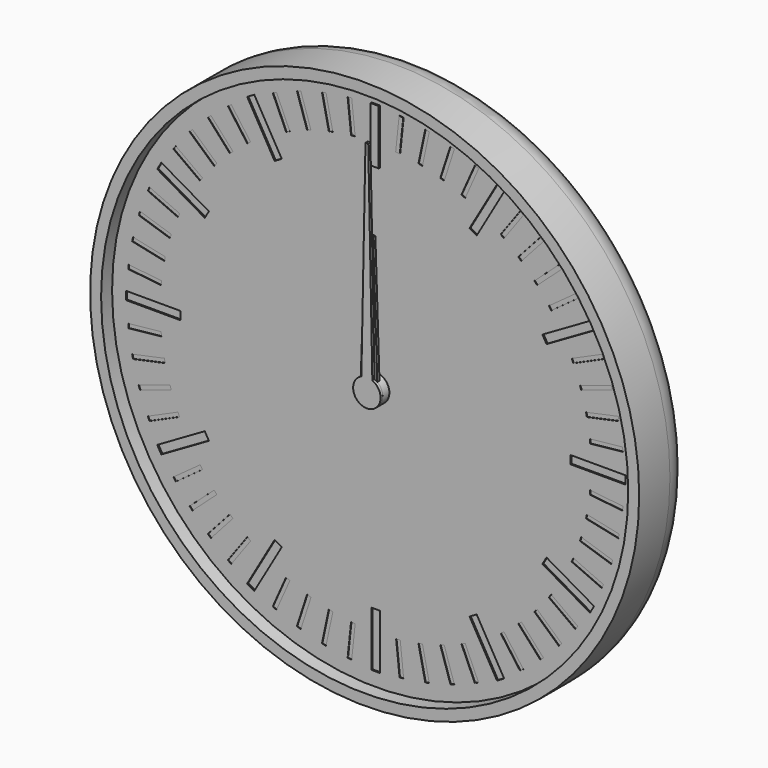
from build123d import *

# Parameters (mm, degrees)
F0_R      = 100
F1_DEPTH  = 24
F2_R      = 10
F3_T      = -4
F4_R      = 5
F4_R_2    = 3
F5_DEPTH  = 2
F6_DEPTH  = 19
F7_DEPTH  = 8
F9_DEPTH  = 4
F11_DEPTH = 4
F12_R     = 5
F12_R_2   = 3
F13_DEPTH = 2
F14_R     = 3
F15_DEPTH = 4
F17_DEPTH = 4
F18_R     = 3
F19_DEPTH = 2
F20_R     = 98
F20_R_2   = 5
F21_DEPTH = 1
F23_R     = 5
F23_R_2   = 3
F24_DEPTH = 2
F25_W     = 3
F25_H     = 20
F25_W_2   = 20
F25_H_2   = 3
F26_DEPTH = 0.5
F27_W     = 1.5
F27_H     = 12
F27_W_2   = 12
F27_H_2   = 1.5
F28_DEPTH = 0.2
F29_DEPTH = 1
F30_DEPTH = 0.4
F31_R     = 5
F31_R_2   = 3
F32_DEPTH = 5
F33_R     = 3
F34_DEPTH = 1
F36_DEPTH = 1


with BuildPart() as f1:
    # F0 (on Front) → F1 (new body)
    with BuildSketch(Plane.XZ):
        Circle(F0_R)
    extrude(amount=F1_DEPTH)

    # F2
    f2_edges = [f1.edges().sort_by_distance(p)[0] for p in [
        (-100, 0, 0),
    ]]
    fillet(f2_edges, radius=F2_R)

    # F3
    f3_openings = [f1.faces().sort_by_distance(p)[0] for p in [
        (0, -24, 0),
    ]]
    offset(amount=F3_T, openings=f3_openings)

    # F4 (on face) → F5 (join)
    with BuildSketch(Plane.XZ.offset(4)):
        Circle(F4_R)
        Circle(F4_R_2, mode=Mode.SUBTRACT)
        with Locations((40, 0)):
            Circle(F4_R)
        with Locations((40, 0)):
            Circle(F4_R_2, mode=Mode.SUBTRACT)
    extrude(amount=F5_DEPTH)


with BuildPart() as f6:
    # F6 (new): a face of the model
    f6_faces = [f1.part.faces().sort_by_distance(p)[0] for p in [
        (0, -4, 0),
    ]]
    extrude(f6_faces, amount=F6_DEPTH)

    # F8 (on face) → F9 (join)
    with BuildSketch(Plane.XZ.offset(6)):
        with BuildLine():
            ThreePointArc((9.2729637667, -1.3794085621), (9.3494561423, -0.6915886375), (9.375, 0))
            ThreePointArc((9.375, 0), (9.3494561423, 0.6915886375), (9.2729637667, 1.3794085621))
            ThreePointArc((9.2729637667, 1.3794085621), (8.9161548403, 2.8970343223), (8.3127812852, 4.3345463782))
            ThreePointArc((8.3127812852, 4.3345463782), (7.5845343223, 5.5104867402), (6.6911892658, 6.566476316))
            ThreePointArc((6.6911892658, 6.566476316), (5.5104867402, 7.5845343223), (4.1773988938, 8.3928519278))
            ThreePointArc((4.1773988938, 8.3928519278), (2.8970343223, 8.9161548403), (1.5536078905, 9.2453733036))
            ThreePointArc((1.5536078905, 9.2453733036), (0, 9.375), (-1.5536078905, 9.2453733036))
            ThreePointArc((-1.5536078905, 9.2453733036), (-2.8970343223, 8.9161548403), (-4.1773988938, 8.3928519278))
            ThreePointArc((-4.1773988938, 8.3928519278), (-5.5104867402, 7.5845343223), (-6.6911892658, 6.566476316))
            ThreePointArc((-6.6911892658, 6.566476316), (-7.5845343223, 5.5104867402), (-8.3127812852, 4.3345463782))
            ThreePointArc((-8.3127812852, 4.3345463782), (-8.9161548403, 2.8970343223), (-9.2729637667, 1.3794085621))
            ThreePointArc((-9.2729637667, 1.3794085621), (-9.375, 0), (-9.2729637667, -1.3794085621))
            ThreePointArc((-9.2729637667, -1.3794085621), (-8.9161548403, -2.8970343223), (-8.3127812852, -4.3345463782))
            ThreePointArc((-8.3127812852, -4.3345463782), (-7.5845343223, -5.5104867402), (-6.6911892658, -6.566476316))
            ThreePointArc((-6.6911892658, -6.566476316), (-5.5104867402, -7.5845343223), (-4.1773988938, -8.3928519278))
            ThreePointArc((-4.1773988938, -8.3928519278), (-2.8970343223, -8.9161548403), (-1.5536078905, -9.2453733036))
            ThreePointArc((-1.5536078905, -9.2453733036), (0, -9.375), (1.5536078905, -9.2453733036))
            ThreePointArc((1.5536078905, -9.2453733036), (2.8970343223, -8.9161548403), (4.1773988938, -8.3928519278))
            ThreePointArc((4.1773988938, -8.3928519278), (5.5104867402, -7.5845343223), (6.6911892658, -6.566476316))
            ThreePointArc((6.6911892658, -6.566476316), (7.5845343223, -5.5104867402), (8.3127812852, -4.3345463782))
            ThreePointArc((8.3127812852, -4.3345463782), (8.9161548403, -2.8970343223), (9.2729637667, -1.3794085621))
        make_face()
        with BuildLine():
            ThreePointArc((8.3127812852, 4.3345463782), (8.9161548403, 2.8970343223), (9.2729637667, 1.3794085621))
            Line((9.2729637667, 1.3794085621), (11.1823199426, 2.3946312492))
            Line((11.1823199426, 2.3946312492), (10.8182678729, 3.515068311))
            Line((10.8182678729, 3.515068311), (10.4542158031, 4.6355053728))
            Line((10.4542158031, 4.6355053728), (8.3127812852, 4.3345463782))
        make_face()
        with BuildLine():
            Line((11.1823199426, -2.3946312492), (9.2729637667, -1.3794085621))
            ThreePointArc((9.2729637667, -1.3794085621), (8.9161548403, -2.8970343223), (8.3127812852, -4.3345463782))
            Line((8.3127812852, -4.3345463782), (10.4542158031, -4.6355053728))
            Line((10.4542158031, -4.6355053728), (10.8182678729, -3.515068311))
            Line((10.8182678729, -3.515068311), (11.1823199426, -2.3946312492))
        make_face()
        with BuildLine():
            ThreePointArc((4.1773988938, 8.3928519278), (5.5104867402, 7.5845343223), (6.6911892658, 6.566476316))
            Line((6.6911892658, 6.566476316), (7.6391579371, 8.5101001246))
            Line((7.6391579371, 8.5101001246), (6.6860572448, 9.202568311))
            Line((6.6860572448, 9.202568311), (5.7329565525, 9.8950364974))
            Line((5.7329565525, 9.8950364974), (4.1773988938, 8.3928519278))
        make_face()
        with BuildLine():
            Line((7.6391579371, -8.5101001246), (6.6911892658, -6.566476316))
            ThreePointArc((6.6911892658, -6.566476316), (5.5104867402, -7.5845343223), (4.1773988938, -8.3928519278))
            Line((4.1773988938, -8.3928519278), (5.7329565525, -9.8950364974))
            Line((5.7329565525, -9.8950364974), (6.6860572448, -9.202568311))
            Line((6.6860572448, -9.202568311), (7.6391579371, -8.5101001246))
        make_face()
        with BuildLine():
            ThreePointArc((-1.5536078905, 9.2453733036), (0, 9.375), (1.5536078905, 9.2453733036))
            Line((1.5536078905, 9.2453733036), (1.1780972451, 11.375))
            Line((1.1780972451, 11.375), (0, 11.375))
            Line((0, 11.375), (-1.1780972451, 11.375))
            Line((-1.1780972451, 11.375), (-1.5536078905, 9.2453733036))
        make_face()
        with BuildLine():
            Line((1.1780972451, -11.375), (1.5536078905, -9.2453733036))
            ThreePointArc((1.5536078905, -9.2453733036), (0, -9.375), (-1.5536078905, -9.2453733036))
            Line((-1.5536078905, -9.2453733036), (-1.1780972451, -11.375))
            Line((-1.1780972451, -11.375), (0, -11.375))
            Line((0, -11.375), (1.1780972451, -11.375))
        make_face()
        with BuildLine():
            ThreePointArc((-6.6911892658, 6.566476316), (-5.5104867402, 7.5845343223), (-4.1773988938, 8.3928519278))
            Line((-4.1773988938, 8.3928519278), (-5.7329565525, 9.8950364974))
            Line((-5.7329565525, 9.8950364974), (-6.6860572448, 9.202568311))
            Line((-6.6860572448, 9.202568311), (-7.6391579371, 8.5101001246))
            Line((-7.6391579371, 8.5101001246), (-6.6911892658, 6.566476316))
        make_face()
        with BuildLine():
            Line((-5.7329565525, -9.8950364974), (-4.1773988938, -8.3928519278))
            ThreePointArc((-4.1773988938, -8.3928519278), (-5.5104867402, -7.5845343223), (-6.6911892658, -6.566476316))
            Line((-6.6911892658, -6.566476316), (-7.6391579371, -8.5101001246))
            Line((-7.6391579371, -8.5101001246), (-6.6860572448, -9.202568311))
            Line((-6.6860572448, -9.202568311), (-5.7329565525, -9.8950364974))
        make_face()
        with BuildLine():
            ThreePointArc((-9.2729637667, 1.3794085621), (-8.9161548403, 2.8970343223), (-8.3127812852, 4.3345463782))
            Line((-8.3127812852, 4.3345463782), (-10.4542158031, 4.6355053728))
            Line((-10.4542158031, 4.6355053728), (-10.8182678729, 3.515068311))
            Line((-10.8182678729, 3.515068311), (-11.1823199426, 2.3946312492))
            Line((-11.1823199426, 2.3946312492), (-9.2729637667, 1.3794085621))
        make_face()
        with BuildLine():
            Line((-10.4542158031, -4.6355053728), (-8.3127812852, -4.3345463782))
            ThreePointArc((-8.3127812852, -4.3345463782), (-8.9161548403, -2.8970343223), (-9.2729637667, -1.3794085621))
            Line((-9.2729637667, -1.3794085621), (-11.1823199426, -2.3946312492))
            Line((-11.1823199426, -2.3946312492), (-10.8182678729, -3.515068311))
            Line((-10.8182678729, -3.515068311), (-10.4542158031, -4.6355053728))
        make_face()
    extrude(amount=F9_DEPTH)

    # F35 (on face) → F36 (join)
    with BuildSketch(Plane.XZ.offset(23)):
        with BuildLine():
            ThreePointArc((-2, 4.582575695), (-2.7386127875, -4.1833001327), (5, 0))
            ThreePointArc((5, 0), (4.1833001327, 2.7386127875), (2, 4.582575695))
            ThreePointArc((2, 4.582575695), (0, 5), (-2, 4.582575695))
        make_face()
        with BuildLine():
            ThreePointArc((-2, 4.582575695), (0, 5), (2, 4.582575695))
            Line((2, 4.582575695), (0.5, 80))
            Line((0.5, 80), (0, 80))
            Line((0, 80), (-0.5, 80))
            Line((-0.5, 80), (-2, 4.582575695))
        make_face()
    extrude(amount=-F36_DEPTH)


with BuildPart() as f7:
    # F7 (new): a face of the model
    f7_faces = [f1.part.faces().sort_by_distance(p)[0] for p in [
        (40, -4, 0),
    ]]
    extrude(f7_faces, amount=F7_DEPTH)

    # F10 (on face) → F11 (join)
    with BuildSketch(Plane.XZ.offset(6)):
        with BuildLine():
            ThreePointArc((68.0829066802, -1.5381733945), (68.1144747006, -0.7693746225), (68.125, 0))
            ThreePointArc((68.125, 0), (68.1144747006, 0.7693746225), (68.0829066802, 1.5381733945))
            ThreePointArc((68.0829066802, 1.5381733945), (67.9709283072, 2.9398630294), (67.7890320221, 4.3342039956))
            ThreePointArc((67.7890320221, 4.3342039956), (67.5104012706, 5.8475163042), (67.1494235596, 7.3433252263))
            ThreePointArc((67.1494235596, 7.3433252263), (66.7484645208, 8.6911029668), (66.280643318, 10.0171558733))
            ThreePointArc((66.280643318, 10.0171558733), (65.6934659962, 11.4394680865), (65.0293803521, 12.8275385085))
            ThreePointArc((65.0293803521, 12.8275385085), (64.3569644814, 14.0625), (63.6236643925, 15.2623099717))
            ThreePointArc((63.6236643925, 15.2623099717), (62.7536029668, 16.5314602207), (61.815433119, 17.7511268046))
            ThreePointArc((61.815433119, 17.7511268046), (60.9009482166, 18.8192983038), (59.934217974, 19.8404278876))
            ThreePointArc((59.934217974, 19.8404278876), (58.8192983038, 20.9009482166), (57.6480467764, 21.8989056799))
            ThreePointArc((57.6480467764, 21.8989056799), (56.5314602207, 22.7536029668), (55.3735505752, 23.5514238999))
            ThreePointArc((55.3735505752, 23.5514238999), (54.0625, 24.3569644814), (52.709356105, 25.0895972944))
            ThreePointArc((52.709356105, 25.0895972944), (51.4394680865, 25.6934659962), (50.1409852457, 26.2331096755))
            ThreePointArc((50.1409852457, 26.2331096755), (48.6911029668, 26.7484645208), (47.2152055856, 27.1837531139))
            ThreePointArc((47.2152055856, 27.1837531139), (45.8475163042, 27.5104012706), (44.4652101991, 27.7682826779))
            ThreePointArc((44.4652101991, 27.7682826779), (42.9398630294, 27.9709283072), (41.4057159597, 28.0898484802))
            ThreePointArc((41.4057159597, 28.0898484802), (40, 28.125), (38.5942840403, 28.0898484802))
            ThreePointArc((38.5942840403, 28.0898484802), (37.0601369706, 27.9709283072), (35.5347898009, 27.7682826779))
            ThreePointArc((35.5347898009, 27.7682826779), (34.1524836958, 27.5104012706), (32.7847944144, 27.1837531139))
            ThreePointArc((32.7847944144, 27.1837531139), (31.3088970332, 26.7484645208), (29.8590147543, 26.2331096755))
            ThreePointArc((29.8590147543, 26.2331096755), (28.5605319135, 25.6934659962), (27.290643895, 25.0895972944))
            ThreePointArc((27.290643895, 25.0895972944), (25.9375, 24.3569644814), (24.6264494248, 23.5514238999))
            ThreePointArc((24.6264494248, 23.5514238999), (23.4685397793, 22.7536029668), (22.3519532236, 21.8989056799))
            ThreePointArc((22.3519532236, 21.8989056799), (21.1807016962, 20.9009482166), (20.065782026, 19.8404278876))
            ThreePointArc((20.065782026, 19.8404278876), (19.0990517834, 18.8192983038), (18.184566881, 17.7511268046))
            ThreePointArc((18.184566881, 17.7511268046), (17.2463970332, 16.5314602207), (16.3763356075, 15.2623099717))
            ThreePointArc((16.3763356075, 15.2623099717), (15.6430355186, 14.0625), (14.9706196479, 12.8275385085))
            ThreePointArc((14.9706196479, 12.8275385085), (14.3065340038, 11.4394680865), (13.719356682, 10.0171558733))
            ThreePointArc((13.719356682, 10.0171558733), (13.2515354792, 8.6911029668), (12.8505764404, 7.3433252263))
            ThreePointArc((12.8505764404, 7.3433252263), (12.4895987294, 5.8475163042), (12.2109679779, 4.3342039956))
            ThreePointArc((12.2109679779, 4.3342039956), (12.0290716928, 2.9398630294), (11.9170933198, 1.5381733945))
            ThreePointArc((11.9170933198, 1.5381733945), (11.875, 0), (11.9170933198, -1.5381733945))
            ThreePointArc((11.9170933198, -1.5381733945), (12.0290716928, -2.9398630294), (12.2109679779, -4.3342039956))
            ThreePointArc((12.2109679779, -4.3342039956), (12.4895987294, -5.8475163042), (12.8505764404, -7.3433252263))
            ThreePointArc((12.8505764404, -7.3433252263), (13.2515354792, -8.6911029668), (13.719356682, -10.0171558733))
            ThreePointArc((13.719356682, -10.0171558733), (14.3065340038, -11.4394680865), (14.9706196479, -12.8275385085))
            ThreePointArc((14.9706196479, -12.8275385085), (15.6430355186, -14.0625), (16.3763356075, -15.2623099717))
            ThreePointArc((16.3763356075, -15.2623099717), (17.2463970332, -16.5314602207), (18.184566881, -17.7511268046))
            ThreePointArc((18.184566881, -17.7511268046), (19.0990517834, -18.8192983038), (20.065782026, -19.8404278876))
            ThreePointArc((20.065782026, -19.8404278876), (21.1807016962, -20.9009482166), (22.3519532236, -21.8989056799))
            ThreePointArc((22.3519532236, -21.8989056799), (23.4685397793, -22.7536029668), (24.6264494248, -23.5514238999))
            ThreePointArc((24.6264494248, -23.5514238999), (25.9375, -24.3569644814), (27.290643895, -25.0895972944))
            ThreePointArc((27.290643895, -25.0895972944), (28.5605319135, -25.6934659962), (29.8590147543, -26.2331096755))
            ThreePointArc((29.8590147543, -26.2331096755), (31.3088970332, -26.7484645208), (32.7847944144, -27.1837531139))
            ThreePointArc((32.7847944144, -27.1837531139), (34.1524836958, -27.5104012706), (35.5347898009, -27.7682826779))
            ThreePointArc((35.5347898009, -27.7682826779), (37.0601369706, -27.9709283072), (38.5942840403, -28.0898484802))
            ThreePointArc((38.5942840403, -28.0898484802), (40, -28.125), (41.4057159597, -28.0898484802))
            ThreePointArc((41.4057159597, -28.0898484802), (42.9398630294, -27.9709283072), (44.4652101991, -27.7682826779))
            ThreePointArc((44.4652101991, -27.7682826779), (45.8475163042, -27.5104012706), (47.2152055856, -27.1837531139))
            ThreePointArc((47.2152055856, -27.1837531139), (48.6911029668, -26.7484645208), (50.1409852457, -26.2331096755))
            ThreePointArc((50.1409852457, -26.2331096755), (51.4394680865, -25.6934659962), (52.709356105, -25.0895972944))
            ThreePointArc((52.709356105, -25.0895972944), (54.0625, -24.3569644814), (55.3735505752, -23.5514238999))
            ThreePointArc((55.3735505752, -23.5514238999), (56.5314602207, -22.7536029668), (57.6480467764, -21.8989056799))
            ThreePointArc((57.6480467764, -21.8989056799), (58.8192983038, -20.9009482166), (59.934217974, -19.8404278876))
            ThreePointArc((59.934217974, -19.8404278876), (60.9009482166, -18.8192983038), (61.815433119, -17.7511268046))
            ThreePointArc((61.815433119, -17.7511268046), (62.7536029668, -16.5314602207), (63.6236643925, -15.2623099717))
            ThreePointArc((63.6236643925, -15.2623099717), (64.3569644814, -14.0625), (65.0293803521, -12.8275385085))
            ThreePointArc((65.0293803521, -12.8275385085), (65.6934659962, -11.4394680865), (66.280643318, -10.0171558733))
            ThreePointArc((66.280643318, -10.0171558733), (66.7484645208, -8.6911029668), (67.1494235596, -7.3433252263))
            ThreePointArc((67.1494235596, -7.3433252263), (67.5104012706, -5.8475163042), (67.7890320221, -4.3342039956))
            ThreePointArc((67.7890320221, -4.3342039956), (67.9709283072, -2.9398630294), (68.0829066802, -1.5381733945))
        make_face()
        with BuildLine():
            ThreePointArc((68.0829066802, 1.5381733945), (68.1144747006, 0.7693746225), (68.125, 0))
            ThreePointArc((68.125, 0), (68.1144747006, -0.7693746225), (68.0829066802, -1.5381733945))
            Line((68.0829066802, -1.5381733945), (70.125, -1.1780972451))
            Line((70.125, -1.1780972451), (70.125, 0))
            Line((70.125, 0), (70.125, 1.1780972451))
            Line((70.125, 1.1780972451), (68.0829066802, 1.5381733945))
        make_face()
        with BuildLine():
            ThreePointArc((67.1494235596, 7.3433252263), (67.5104012706, 5.8475163042), (67.7890320221, 4.3342039956))
            Line((67.7890320221, 4.3342039956), (69.7116366623, 5.1109866922))
            Line((69.7116366623, 5.1109866922), (69.4666964721, 6.2633396859))
            Line((69.4666964721, 6.2633396859), (69.2217562819, 7.4156926796))
            Line((69.2217562819, 7.4156926796), (67.1494235596, 7.3433252263))
        make_face()
        with BuildLine():
            Line((69.7116366623, -5.1109866922), (67.7890320221, -4.3342039956))
            ThreePointArc((67.7890320221, -4.3342039956), (67.5104012706, -5.8475163042), (67.1494235596, -7.3433252263))
            Line((67.1494235596, -7.3433252263), (69.2217562819, -7.4156926796))
            Line((69.2217562819, -7.4156926796), (69.4666964721, -6.2633396859))
            Line((69.4666964721, -6.2633396859), (69.7116366623, -5.1109866922))
        make_face()
        with BuildLine():
            ThreePointArc((65.0293803521, 12.8275385085), (65.6934659962, 11.4394680865), (66.280643318, 10.0171558733))
            Line((66.280643318, 10.0171558733), (67.9997322302, 11.1766959857))
            Line((67.9997322302, 11.1766959857), (67.5205569115, 12.2529413727))
            Line((67.5205569115, 12.2529413727), (67.0413815928, 13.3291867596))
            Line((67.0413815928, 13.3291867596), (65.0293803521, 12.8275385085))
        make_face()
        with BuildLine():
            Line((67.9997322302, -11.1766959857), (66.280643318, -10.0171558733))
            ThreePointArc((66.280643318, -10.0171558733), (65.6934659962, -11.4394680865), (65.0293803521, -12.8275385085))
            Line((65.0293803521, -12.8275385085), (67.0413815928, -13.3291867596))
            Line((67.0413815928, -13.3291867596), (67.5205569115, -12.2529413727))
            Line((67.5205569115, -12.2529413727), (67.9997322302, -11.1766959857))
        make_face()
        with BuildLine():
            ThreePointArc((61.815433119, 17.7511268046), (62.7536029668, 16.5314602207), (63.6236643925, 15.2623099717))
            Line((63.6236643925, 15.2623099717), (65.064105142, 16.753930033))
            Line((65.064105142, 16.753930033), (64.3716369555, 17.7070307253))
            Line((64.3716369555, 17.7070307253), (63.6791687691, 18.6601314176))
            Line((63.6791687691, 18.6601314176), (61.815433119, 17.7511268046))
        make_face()
        with BuildLine():
            Line((65.064105142, -16.753930033), (63.6236643925, -15.2623099717))
            ThreePointArc((63.6236643925, -15.2623099717), (62.7536029668, -16.5314602207), (61.815433119, -17.7511268046))
            Line((61.815433119, -17.7511268046), (63.6791687691, -18.6601314176))
            Line((63.6791687691, -18.6601314176), (64.3716369555, -17.7070307253))
            Line((64.3716369555, -17.7070307253), (65.064105142, -16.753930033))
        make_face()
        with BuildLine():
            ThreePointArc((57.6480467764, 21.8989056799), (58.8192983038, 20.9009482166), (59.934217974, 19.8404278876))
            Line((59.934217974, 19.8404278876), (61.0330563882, 21.5989369435))
            Line((61.0330563882, 21.5989369435), (60.1575595166, 22.3872378675))
            Line((60.1575595166, 22.3872378675), (59.282062645, 23.1755387915))
            Line((59.282062645, 23.1755387915), (57.6480467764, 21.8989056799))
        make_face()
        with BuildLine():
            Line((61.0330563882, -21.5989369435), (59.934217974, -19.8404278876))
            ThreePointArc((59.934217974, -19.8404278876), (58.8192983038, -20.9009482166), (57.6480467764, -21.8989056799))
            Line((57.6480467764, -21.8989056799), (59.282062645, -23.1755387915))
            Line((59.282062645, -23.1755387915), (60.1575595166, -22.3872378675))
            Line((60.1575595166, -22.3872378675), (61.0330563882, -21.5989369435))
        make_face()
        with BuildLine():
            ThreePointArc((52.709356105, 25.0895972944), (54.0625, 24.3569644814), (55.3735505752, 23.5514238999))
            Line((55.3735505752, 23.5514238999), (56.0827621424, 25.4999666665))
            Line((56.0827621424, 25.4999666665), (55.0625, 26.089015289))
            Line((55.0625, 26.089015289), (54.0422378576, 26.6780639116))
            Line((54.0422378576, 26.6780639116), (52.709356105, 25.0895972944))
        make_face()
        with BuildLine():
            Line((56.0827621424, -25.4999666665), (55.3735505752, -23.5514238999))
            ThreePointArc((55.3735505752, -23.5514238999), (54.0625, -24.3569644814), (52.709356105, -25.0895972944))
            Line((52.709356105, -25.0895972944), (54.0422378576, -26.6780639116))
            Line((54.0422378576, -26.6780639116), (55.0625, -26.089015289))
            Line((55.0625, -26.089015289), (56.0827621424, -25.4999666665))
        make_face()
        with BuildLine():
            ThreePointArc((47.2152055856, 27.1837531139), (48.6911029668, 26.7484645208), (50.1409852457, 26.2331096755))
            Line((50.1409852457, 26.2331096755), (50.4295740173, 28.2865254836))
            Line((50.4295740173, 28.2865254836), (49.3091369555, 28.6505775534))
            Line((49.3091369555, 28.6505775534), (48.1886998938, 29.0146296232))
            Line((48.1886998938, 29.0146296232), (47.2152055856, 27.1837531139))
        make_face()
        with BuildLine():
            Line((50.4295740173, -28.2865254836), (50.1409852457, -26.2331096755))
            ThreePointArc((50.1409852457, -26.2331096755), (48.6911029668, -26.7484645208), (47.2152055856, -27.1837531139))
            Line((47.2152055856, -27.1837531139), (48.1886998938, -29.0146296232))
            Line((48.1886998938, -29.0146296232), (49.3091369555, -28.6505775534))
            Line((49.3091369555, -28.6505775534), (50.4295740173, -28.2865254836))
        make_face()
        with BuildLine():
            ThreePointArc((41.4057159597, 28.0898484802), (42.9398630294, 27.9709283072), (44.4652101991, 27.7682826779))
            Line((44.4652101991, 27.7682826779), (44.3205634611, 29.8368274034))
            Line((44.3205634611, 29.8368274034), (43.1489199559, 29.959972098))
            Line((43.1489199559, 29.959972098), (41.9772764508, 30.0831167926))
            Line((41.9772764508, 30.0831167926), (41.4057159597, 28.0898484802))
        make_face()
        with BuildLine():
            Line((44.3205634611, -29.8368274034), (44.4652101991, -27.7682826779))
            ThreePointArc((44.4652101991, -27.7682826779), (42.9398630294, -27.9709283072), (41.4057159597, -28.0898484802))
            Line((41.4057159597, -28.0898484802), (41.9772764508, -30.0831167926))
            Line((41.9772764508, -30.0831167926), (43.1489199559, -29.959972098))
            Line((43.1489199559, -29.959972098), (44.3205634611, -29.8368274034))
        make_face()
        with BuildLine():
            ThreePointArc((35.5347898009, 27.7682826779), (37.0601369706, 27.9709283072), (38.5942840403, 28.0898484802))
            Line((38.5942840403, 28.0898484802), (38.0227235492, 30.0831167926))
            Line((38.0227235492, 30.0831167926), (36.8510800441, 29.959972098))
            Line((36.8510800441, 29.959972098), (35.6794365389, 29.8368274034))
            Line((35.6794365389, 29.8368274034), (35.5347898009, 27.7682826779))
        make_face()
        with BuildLine():
            Line((38.0227235492, -30.0831167926), (38.5942840403, -28.0898484802))
            ThreePointArc((38.5942840403, -28.0898484802), (37.0601369706, -27.9709283072), (35.5347898009, -27.7682826779))
            Line((35.5347898009, -27.7682826779), (35.6794365389, -29.8368274034))
            Line((35.6794365389, -29.8368274034), (36.8510800441, -29.959972098))
            Line((36.8510800441, -29.959972098), (38.0227235492, -30.0831167926))
        make_face()
        with BuildLine():
            ThreePointArc((29.8590147543, 26.2331096755), (31.3088970332, 26.7484645208), (32.7847944144, 27.1837531139))
            Line((32.7847944144, 27.1837531139), (31.8113001062, 29.0146296232))
            Line((31.8113001062, 29.0146296232), (30.6908630445, 28.6505775534))
            Line((30.6908630445, 28.6505775534), (29.5704259827, 28.2865254836))
            Line((29.5704259827, 28.2865254836), (29.8590147543, 26.2331096755))
        make_face()
        with BuildLine():
            Line((31.8113001062, -29.0146296232), (32.7847944144, -27.1837531139))
            ThreePointArc((32.7847944144, -27.1837531139), (31.3088970332, -26.7484645208), (29.8590147543, -26.2331096755))
            Line((29.8590147543, -26.2331096755), (29.5704259827, -28.2865254836))
            Line((29.5704259827, -28.2865254836), (30.6908630445, -28.6505775534))
            Line((30.6908630445, -28.6505775534), (31.8113001062, -29.0146296232))
        make_face()
        with BuildLine():
            ThreePointArc((24.6264494248, 23.5514238999), (25.9375, 24.3569644814), (27.290643895, 25.0895972944))
            Line((27.290643895, 25.0895972944), (25.9577621424, 26.6780639116))
            Line((25.9577621424, 26.6780639116), (24.9375, 26.089015289))
            Line((24.9375, 26.089015289), (23.9172378576, 25.4999666665))
            Line((23.9172378576, 25.4999666665), (24.6264494248, 23.5514238999))
        make_face()
        with BuildLine():
            Line((25.9577621424, -26.6780639116), (27.290643895, -25.0895972944))
            ThreePointArc((27.290643895, -25.0895972944), (25.9375, -24.3569644814), (24.6264494248, -23.5514238999))
            Line((24.6264494248, -23.5514238999), (23.9172378576, -25.4999666665))
            Line((23.9172378576, -25.4999666665), (24.9375, -26.089015289))
            Line((24.9375, -26.089015289), (25.9577621424, -26.6780639116))
        make_face()
        with BuildLine():
            ThreePointArc((20.065782026, 19.8404278876), (21.1807016962, 20.9009482166), (22.3519532236, 21.8989056799))
            Line((22.3519532236, 21.8989056799), (20.717937355, 23.1755387915))
            Line((20.717937355, 23.1755387915), (19.8424404834, 22.3872378675))
            Line((19.8424404834, 22.3872378675), (18.9669436118, 21.5989369435))
            Line((18.9669436118, 21.5989369435), (20.065782026, 19.8404278876))
        make_face()
        with BuildLine():
            Line((20.717937355, -23.1755387915), (22.3519532236, -21.8989056799))
            ThreePointArc((22.3519532236, -21.8989056799), (21.1807016962, -20.9009482166), (20.065782026, -19.8404278876))
            Line((20.065782026, -19.8404278876), (18.9669436118, -21.5989369435))
            Line((18.9669436118, -21.5989369435), (19.8424404834, -22.3872378675))
            Line((19.8424404834, -22.3872378675), (20.717937355, -23.1755387915))
        make_face()
        with BuildLine():
            ThreePointArc((16.3763356075, 15.2623099717), (17.2463970332, 16.5314602207), (18.184566881, 17.7511268046))
            Line((18.184566881, 17.7511268046), (16.3208312309, 18.6601314176))
            Line((16.3208312309, 18.6601314176), (15.6283630445, 17.7070307253))
            Line((15.6283630445, 17.7070307253), (14.935894858, 16.753930033))
            Line((14.935894858, 16.753930033), (16.3763356075, 15.2623099717))
        make_face()
        with BuildLine():
            Line((16.3208312309, -18.6601314176), (18.184566881, -17.7511268046))
            ThreePointArc((18.184566881, -17.7511268046), (17.2463970332, -16.5314602207), (16.3763356075, -15.2623099717))
            Line((16.3763356075, -15.2623099717), (14.935894858, -16.753930033))
            Line((14.935894858, -16.753930033), (15.6283630445, -17.7070307253))
            Line((15.6283630445, -17.7070307253), (16.3208312309, -18.6601314176))
        make_face()
        with BuildLine():
            ThreePointArc((13.719356682, 10.0171558733), (14.3065340038, 11.4394680865), (14.9706196479, 12.8275385085))
            Line((14.9706196479, 12.8275385085), (12.9586184072, 13.3291867596))
            Line((12.9586184072, 13.3291867596), (12.4794430885, 12.2529413727))
            Line((12.4794430885, 12.2529413727), (12.0002677698, 11.1766959857))
            Line((12.0002677698, 11.1766959857), (13.719356682, 10.0171558733))
        make_face()
        with BuildLine():
            Line((12.9586184072, -13.3291867596), (14.9706196479, -12.8275385085))
            ThreePointArc((14.9706196479, -12.8275385085), (14.3065340038, -11.4394680865), (13.719356682, -10.0171558733))
            Line((13.719356682, -10.0171558733), (12.0002677698, -11.1766959857))
            Line((12.0002677698, -11.1766959857), (12.4794430885, -12.2529413727))
            Line((12.4794430885, -12.2529413727), (12.9586184072, -13.3291867596))
        make_face()
        with BuildLine():
            ThreePointArc((12.2109679779, 4.3342039956), (12.4895987294, 5.8475163042), (12.8505764404, 7.3433252263))
            Line((12.8505764404, 7.3433252263), (10.7782437181, 7.4156926796))
            Line((10.7782437181, 7.4156926796), (10.5333035279, 6.2633396859))
            Line((10.5333035279, 6.2633396859), (10.2883633377, 5.1109866922))
            Line((10.2883633377, 5.1109866922), (12.2109679779, 4.3342039956))
        make_face()
        with BuildLine():
            Line((10.7782437181, -7.4156926796), (12.8505764404, -7.3433252263))
            ThreePointArc((12.8505764404, -7.3433252263), (12.4895987294, -5.8475163042), (12.2109679779, -4.3342039956))
            Line((12.2109679779, -4.3342039956), (10.2883633377, -5.1109866922))
            Line((10.2883633377, -5.1109866922), (10.5333035279, -6.2633396859))
            Line((10.5333035279, -6.2633396859), (10.7782437181, -7.4156926796))
        make_face()
        with BuildLine():
            ThreePointArc((11.9170933198, -1.5381733945), (11.875, 0), (11.9170933198, 1.5381733945))
            Line((11.9170933198, 1.5381733945), (9.875, 1.1780972451))
            Line((9.875, 1.1780972451), (9.875, 0))
            Line((9.875, 0), (9.875, -1.1780972451))
            Line((9.875, -1.1780972451), (11.9170933198, -1.5381733945))
        make_face()
    extrude(amount=F11_DEPTH)

    # F16 (on face) → F17 (join)
    with BuildSketch(Plane.XZ.offset(12)):
        with BuildLine():
            ThreePointArc((47.4288750323, -1.0304444454), (47.4821976298, -0.5164480894), (47.5, 0))
            ThreePointArc((47.5, 0), (47.4821976298, 0.5164480894), (47.4288750323, 1.0304444454))
            ThreePointArc((47.4288750323, 1.0304444454), (47.1329238722, 2.3176274578), (46.6157661985, 3.532936117))
            ThreePointArc((46.6157661985, 3.532936117), (46.0676274578, 4.4083893922), (45.4044061018, 5.2002302532))
            ThreePointArc((45.4044061018, 5.2002302532), (44.4083893922, 6.0676274578), (43.2756595386, 6.7468551628))
            ThreePointArc((43.2756595386, 6.7468551628), (42.3176274578, 7.1329238722), (41.3156377295, 7.3837048536))
            ThreePointArc((41.3156377295, 7.3837048536), (40, 7.5), (38.6843622705, 7.3837048536))
            ThreePointArc((38.6843622705, 7.3837048536), (37.6823725422, 7.1329238722), (36.7243404614, 6.7468551628))
            ThreePointArc((36.7243404614, 6.7468551628), (35.5916106078, 6.0676274578), (34.5955938982, 5.2002302532))
            ThreePointArc((34.5955938982, 5.2002302532), (33.9323725422, 4.4083893922), (33.3842338015, 3.532936117))
            ThreePointArc((33.3842338015, 3.532936117), (32.8670761278, 2.3176274578), (32.5711249677, 1.0304444454))
            ThreePointArc((32.5711249677, 1.0304444454), (32.5, 0), (32.5711249677, -1.0304444454))
            ThreePointArc((32.5711249677, -1.0304444454), (32.8670761278, -2.3176274578), (33.3842338015, -3.532936117))
            ThreePointArc((33.3842338015, -3.532936117), (33.9323725422, -4.4083893922), (34.5955938982, -5.2002302532))
            ThreePointArc((34.5955938982, -5.2002302532), (35.5916106078, -6.0676274578), (36.7243404614, -6.7468551628))
            ThreePointArc((36.7243404614, -6.7468551628), (37.6823725422, -7.1329238722), (38.6843622705, -7.3837048536))
            ThreePointArc((38.6843622705, -7.3837048536), (40, -7.5), (41.3156377295, -7.3837048536))
            ThreePointArc((41.3156377295, -7.3837048536), (42.3176274578, -7.1329238722), (43.2756595386, -6.7468551628))
            ThreePointArc((43.2756595386, -6.7468551628), (44.4083893922, -6.0676274578), (45.4044061018, -5.2002302532))
            ThreePointArc((45.4044061018, -5.2002302532), (46.0676274578, -4.4083893922), (46.6157661985, -3.532936117))
            ThreePointArc((46.6157661985, -3.532936117), (47.1329238722, -2.3176274578), (47.4288750323, -1.0304444454))
        make_face()
        with BuildLine():
            ThreePointArc((46.6157661985, 3.532936117), (47.1329238722, 2.3176274578), (47.4288750323, 1.0304444454))
            Line((47.4288750323, 1.0304444454), (49.3262785606, 2.0393117971))
            Line((49.3262785606, 2.0393117971), (48.743795249, 3.832011096))
            Line((48.743795249, 3.832011096), (46.6157661985, 3.532936117))
        make_face()
        with BuildLine():
            Line((49.3262785606, -2.0393117971), (47.4288750323, -1.0304444454))
            ThreePointArc((47.4288750323, -1.0304444454), (47.1329238722, -2.3176274578), (46.6157661985, -3.532936117))
            Line((46.6157661985, -3.532936117), (48.743795249, -3.832011096))
            Line((48.743795249, -3.832011096), (49.3262785606, -2.0393117971))
        make_face()
        with BuildLine():
            ThreePointArc((43.2756595386, 6.7468551628), (44.4083893922, 6.0676274578), (45.4044061018, 5.2002302532))
            Line((45.4044061018, 5.2002302532), (46.3464404506, 7.1316868974))
            Line((46.3464404506, 7.1316868974), (44.8214793429, 8.2396359957))
            Line((44.8214793429, 8.2396359957), (43.2756595386, 6.7468551628))
        make_face()
        with BuildLine():
            Line((46.3464404506, -7.1316868974), (45.4044061018, -5.2002302532))
            ThreePointArc((45.4044061018, -5.2002302532), (44.4083893922, -6.0676274578), (43.2756595386, -6.7468551628))
            Line((43.2756595386, -6.7468551628), (44.8214793429, -8.2396359957))
            Line((44.8214793429, -8.2396359957), (46.3464404506, -7.1316868974))
        make_face()
        with BuildLine():
            ThreePointArc((38.6843622705, 7.3837048536), (40, 7.5), (41.3156377295, 7.3837048536))
            Line((41.3156377295, 7.3837048536), (40.9424777961, 9.5))
            Line((40.9424777961, 9.5), (39.0575222039, 9.5))
            Line((39.0575222039, 9.5), (38.6843622705, 7.3837048536))
        make_face()
        with BuildLine():
            Line((40.9424777961, -9.5), (41.3156377295, -7.3837048536))
            ThreePointArc((41.3156377295, -7.3837048536), (40, -7.5), (38.6843622705, -7.3837048536))
            Line((38.6843622705, -7.3837048536), (39.0575222039, -9.5))
            Line((39.0575222039, -9.5), (40.9424777961, -9.5))
        make_face()
        with BuildLine():
            ThreePointArc((34.5955938982, 5.2002302532), (35.5916106078, 6.0676274578), (36.7243404614, 6.7468551628))
            Line((36.7243404614, 6.7468551628), (35.1785206571, 8.2396359957))
            Line((35.1785206571, 8.2396359957), (33.6535595494, 7.1316868974))
            Line((33.6535595494, 7.1316868974), (34.5955938982, 5.2002302532))
        make_face()
        with BuildLine():
            Line((35.1785206571, -8.2396359957), (36.7243404614, -6.7468551628))
            ThreePointArc((36.7243404614, -6.7468551628), (35.5916106078, -6.0676274578), (34.5955938982, -5.2002302532))
            Line((34.5955938982, -5.2002302532), (33.6535595494, -7.1316868974))
            Line((33.6535595494, -7.1316868974), (35.1785206571, -8.2396359957))
        make_face()
        with BuildLine():
            ThreePointArc((32.5711249677, 1.0304444454), (32.8670761278, 2.3176274578), (33.3842338015, 3.532936117))
            Line((33.3842338015, 3.532936117), (31.256204751, 3.832011096))
            Line((31.256204751, 3.832011096), (30.6737214394, 2.0393117971))
            Line((30.6737214394, 2.0393117971), (32.5711249677, 1.0304444454))
        make_face()
        with BuildLine():
            Line((31.256204751, -3.832011096), (33.3842338015, -3.532936117))
            ThreePointArc((33.3842338015, -3.532936117), (32.8670761278, -2.3176274578), (32.5711249677, -1.0304444454))
            Line((32.5711249677, -1.0304444454), (30.6737214394, -2.0393117971))
            Line((30.6737214394, -2.0393117971), (31.256204751, -3.832011096))
        make_face()
    extrude(amount=F17_DEPTH)

    # F18 (on face) → F19 (join)
    with BuildSketch(Plane.XZ.offset(16)):
        with Locations((40, 0)):
            Circle(F18_R)
    extrude(amount=F19_DEPTH)


with BuildPart() as f13:
    # F12 (on face) → F13 (new body)
    with BuildSketch(Plane.XZ.offset(10)):
        Circle(F12_R)
        Circle(F12_R_2, mode=Mode.SUBTRACT)
    extrude(amount=F13_DEPTH)

    # F14 (on face) → F15 (join)
    with BuildSketch(Plane.XZ.offset(12)):
        with BuildLine():
            ThreePointArc((29.9718156995, -1.3001014101), (29.9929530972, -0.6502034357), (30, 0))
            ThreePointArc((30, 0), (29.9929530972, 0.6502034357), (29.9718156995, 1.3001014101))
            ThreePointArc((29.9718156995, 1.3001014101), (29.907520012, 2.3537728718), (29.8061935814, 3.4045299509))
            ThreePointArc((29.8061935814, 3.4045299509), (29.6306502179, 4.6930339512), (29.3994322443, 5.9727199596))
            ThreePointArc((29.3994322443, 5.9727199596), (29.1710976119, 7.0033609157), (28.9066440563, 8.0253304855))
            ThreePointArc((28.9066440563, 8.0253304855), (28.5316954889, 9.2705098312), (28.1031371961, 10.4982703213))
            ThreePointArc((28.1031371961, 10.4982703213), (27.7163859753, 11.480502971), (27.2953170189, 12.448520749))
            ThreePointArc((27.2953170189, 12.448520749), (26.7301957257, 13.6197149922), (26.1148496411, 14.765318426))
            ThreePointArc((26.1148496411, 14.765318426), (25.5792049306, 15.6749569415), (25.0118886885, 16.5651871174))
            ThreePointArc((25.0118886885, 16.5651871174), (24.2705098312, 17.6335575688), (23.4835278178, 18.6687953878))
            ThreePointArc((23.4835278178, 18.6687953878), (22.812178968, 19.4834414499), (22.1125846489, 20.2739636023))
            ThreePointArc((22.1125846489, 20.2739636023), (21.2132034356, 21.2132034356), (20.2739636023, 22.1125846489))
            ThreePointArc((20.2739636023, 22.1125846489), (19.4834414499, 22.812178968), (18.6687953878, 23.4835278178))
            ThreePointArc((18.6687953878, 23.4835278178), (17.6335575688, 24.2705098312), (16.5651871174, 25.0118886885))
            ThreePointArc((16.5651871174, 25.0118886885), (15.6749569415, 25.5792049306), (14.765318426, 26.1148496411))
            ThreePointArc((14.765318426, 26.1148496411), (13.6197149922, 26.7301957257), (12.448520749, 27.2953170189))
            ThreePointArc((12.448520749, 27.2953170189), (11.480502971, 27.7163859753), (10.4982703213, 28.1031371961))
            ThreePointArc((10.4982703213, 28.1031371961), (9.2705098312, 28.5316954889), (8.0253304855, 28.9066440563))
            ThreePointArc((8.0253304855, 28.9066440563), (7.0033609157, 29.1710976119), (5.9727199596, 29.3994322443))
            ThreePointArc((5.9727199596, 29.3994322443), (4.6930339512, 29.6306502179), (3.4045299509, 29.8061935814))
            ThreePointArc((3.4045299509, 29.8061935814), (2.3537728718, 29.907520012), (1.3001014101, 29.9718156995))
            ThreePointArc((1.3001014101, 29.9718156995), (0, 30), (-1.3001014101, 29.9718156995))
            ThreePointArc((-1.3001014101, 29.9718156995), (-2.3537728718, 29.907520012), (-3.4045299509, 29.8061935814))
            ThreePointArc((-3.4045299509, 29.8061935814), (-4.6930339512, 29.6306502179), (-5.9727199596, 29.3994322443))
            ThreePointArc((-5.9727199596, 29.3994322443), (-7.0033609157, 29.1710976119), (-8.0253304855, 28.9066440563))
            ThreePointArc((-8.0253304855, 28.9066440563), (-9.2705098312, 28.5316954889), (-10.4982703213, 28.1031371961))
            ThreePointArc((-10.4982703213, 28.1031371961), (-11.480502971, 27.7163859753), (-12.448520749, 27.2953170189))
            ThreePointArc((-12.448520749, 27.2953170189), (-13.6197149922, 26.7301957257), (-14.765318426, 26.1148496411))
            ThreePointArc((-14.765318426, 26.1148496411), (-15.6749569415, 25.5792049306), (-16.5651871174, 25.0118886885))
            ThreePointArc((-16.5651871174, 25.0118886885), (-17.6335575688, 24.2705098312), (-18.6687953878, 23.4835278178))
            ThreePointArc((-18.6687953878, 23.4835278178), (-19.4834414499, 22.812178968), (-20.2739636023, 22.1125846489))
            ThreePointArc((-20.2739636023, 22.1125846489), (-21.2132034356, 21.2132034356), (-22.1125846489, 20.2739636023))
            ThreePointArc((-22.1125846489, 20.2739636023), (-22.812178968, 19.4834414499), (-23.4835278178, 18.6687953878))
            ThreePointArc((-23.4835278178, 18.6687953878), (-24.2705098312, 17.6335575688), (-25.0118886885, 16.5651871174))
            ThreePointArc((-25.0118886885, 16.5651871174), (-25.5792049306, 15.6749569415), (-26.1148496411, 14.765318426))
            ThreePointArc((-26.1148496411, 14.765318426), (-26.7301957257, 13.6197149922), (-27.2953170189, 12.448520749))
            ThreePointArc((-27.2953170189, 12.448520749), (-27.7163859753, 11.480502971), (-28.1031371961, 10.4982703213))
            ThreePointArc((-28.1031371961, 10.4982703213), (-28.5316954889, 9.2705098312), (-28.9066440563, 8.0253304855))
            ThreePointArc((-28.9066440563, 8.0253304855), (-29.1710976119, 7.0033609157), (-29.3994322443, 5.9727199596))
            ThreePointArc((-29.3994322443, 5.9727199596), (-29.6306502179, 4.6930339512), (-29.8061935814, 3.4045299509))
            ThreePointArc((-29.8061935814, 3.4045299509), (-29.907520012, 2.3537728718), (-29.9718156995, 1.3001014101))
            ThreePointArc((-29.9718156995, 1.3001014101), (-30, 0), (-29.9718156995, -1.3001014101))
            ThreePointArc((-29.9718156995, -1.3001014101), (-29.907520012, -2.3537728718), (-29.8061935814, -3.4045299509))
            ThreePointArc((-29.8061935814, -3.4045299509), (-29.6306502179, -4.6930339512), (-29.3994322443, -5.9727199596))
            ThreePointArc((-29.3994322443, -5.9727199596), (-29.1710976119, -7.0033609157), (-28.9066440563, -8.0253304855))
            ThreePointArc((-28.9066440563, -8.0253304855), (-28.5316954889, -9.2705098312), (-28.1031371961, -10.4982703213))
            ThreePointArc((-28.1031371961, -10.4982703213), (-27.7163859753, -11.480502971), (-27.2953170189, -12.448520749))
            ThreePointArc((-27.2953170189, -12.448520749), (-26.7301957257, -13.6197149922), (-26.1148496411, -14.765318426))
            ThreePointArc((-26.1148496411, -14.765318426), (-25.5792049306, -15.6749569415), (-25.0118886885, -16.5651871174))
            ThreePointArc((-25.0118886885, -16.5651871174), (-24.2705098312, -17.6335575688), (-23.4835278178, -18.6687953878))
            ThreePointArc((-23.4835278178, -18.6687953878), (-22.812178968, -19.4834414499), (-22.1125846489, -20.2739636023))
            ThreePointArc((-22.1125846489, -20.2739636023), (-21.2132034356, -21.2132034356), (-20.2739636023, -22.1125846489))
            ThreePointArc((-20.2739636023, -22.1125846489), (-19.4834414499, -22.812178968), (-18.6687953878, -23.4835278178))
            ThreePointArc((-18.6687953878, -23.4835278178), (-17.6335575688, -24.2705098312), (-16.5651871174, -25.0118886885))
            ThreePointArc((-16.5651871174, -25.0118886885), (-15.6749569415, -25.5792049306), (-14.765318426, -26.1148496411))
            ThreePointArc((-14.765318426, -26.1148496411), (-13.6197149922, -26.7301957257), (-12.448520749, -27.2953170189))
            ThreePointArc((-12.448520749, -27.2953170189), (-11.480502971, -27.7163859753), (-10.4982703213, -28.1031371961))
            ThreePointArc((-10.4982703213, -28.1031371961), (-9.2705098312, -28.5316954889), (-8.0253304855, -28.9066440563))
            ThreePointArc((-8.0253304855, -28.9066440563), (-7.0033609157, -29.1710976119), (-5.9727199596, -29.3994322443))
            ThreePointArc((-5.9727199596, -29.3994322443), (-4.6930339512, -29.6306502179), (-3.4045299509, -29.8061935814))
            ThreePointArc((-3.4045299509, -29.8061935814), (-2.3537728718, -29.907520012), (-1.3001014101, -29.9718156995))
            ThreePointArc((-1.3001014101, -29.9718156995), (0, -30), (1.3001014101, -29.9718156995))
            ThreePointArc((1.3001014101, -29.9718156995), (2.3537728718, -29.907520012), (3.4045299509, -29.8061935814))
            ThreePointArc((3.4045299509, -29.8061935814), (4.6930339512, -29.6306502179), (5.9727199596, -29.3994322443))
            ThreePointArc((5.9727199596, -29.3994322443), (7.0033609157, -29.1710976119), (8.0253304855, -28.9066440563))
            ThreePointArc((8.0253304855, -28.9066440563), (9.2705098312, -28.5316954889), (10.4982703213, -28.1031371961))
            ThreePointArc((10.4982703213, -28.1031371961), (11.480502971, -27.7163859753), (12.448520749, -27.2953170189))
            ThreePointArc((12.448520749, -27.2953170189), (13.6197149922, -26.7301957257), (14.765318426, -26.1148496411))
            ThreePointArc((14.765318426, -26.1148496411), (15.6749569415, -25.5792049306), (16.5651871174, -25.0118886885))
            ThreePointArc((16.5651871174, -25.0118886885), (17.6335575688, -24.2705098312), (18.6687953878, -23.4835278178))
            ThreePointArc((18.6687953878, -23.4835278178), (19.4834414499, -22.812178968), (20.2739636023, -22.1125846489))
            ThreePointArc((20.2739636023, -22.1125846489), (21.2132034356, -21.2132034356), (22.1125846489, -20.2739636023))
            ThreePointArc((22.1125846489, -20.2739636023), (22.812178968, -19.4834414499), (23.4835278178, -18.6687953878))
            ThreePointArc((23.4835278178, -18.6687953878), (24.2705098312, -17.6335575688), (25.0118886885, -16.5651871174))
            ThreePointArc((25.0118886885, -16.5651871174), (25.5792049306, -15.6749569415), (26.1148496411, -14.765318426))
            ThreePointArc((26.1148496411, -14.765318426), (26.7301957257, -13.6197149922), (27.2953170189, -12.448520749))
            ThreePointArc((27.2953170189, -12.448520749), (27.7163859753, -11.480502971), (28.1031371961, -10.4982703213))
            ThreePointArc((28.1031371961, -10.4982703213), (28.5316954889, -9.2705098312), (28.9066440563, -8.0253304855))
            ThreePointArc((28.9066440563, -8.0253304855), (29.1710976119, -7.0033609157), (29.3994322443, -5.9727199596))
            ThreePointArc((29.3994322443, -5.9727199596), (29.6306502179, -4.6930339512), (29.8061935814, -3.4045299509))
            ThreePointArc((29.8061935814, -3.4045299509), (29.907520012, -2.3537728718), (29.9718156995, -1.3001014101))
        make_face()
        Circle(F14_R, mode=Mode.SUBTRACT)
        with BuildLine():
            ThreePointArc((29.9718156995, 1.3001014101), (29.9929530972, 0.6502034357), (30, 0))
            ThreePointArc((30, 0), (29.9929530972, -0.6502034357), (29.9718156995, -1.3001014101))
            Line((29.9718156995, -1.3001014101), (32, -0.9424777961))
            Line((32, -0.9424777961), (32, 0))
            Line((32, 0), (32, 0.9424777961))
            Line((32, 0.9424777961), (29.9718156995, 1.3001014101))
        make_face()
        with BuildLine():
            ThreePointArc((29.3994322443, 5.9727199596), (29.6306502179, 4.6930339512), (29.8061935814, 3.4045299509))
            Line((29.8061935814, 3.4045299509), (31.7534629089, 4.0750285508))
            Line((31.7534629089, 4.0750285508), (31.606026899, 5.0059028813))
            Line((31.606026899, 5.0059028813), (31.4585908892, 5.9367772117))
            Line((31.4585908892, 5.9367772117), (29.3994322443, 5.9727199596))
        make_face()
        with BuildLine():
            Line((31.7534629089, -4.0750285508), (29.8061935814, -3.4045299509))
            ThreePointArc((29.8061935814, -3.4045299509), (29.6306502179, -4.6930339512), (29.3994322443, -5.9727199596))
            Line((29.3994322443, -5.9727199596), (31.4585908892, -5.9367772117))
            Line((31.4585908892, -5.9367772117), (31.606026899, -5.0059028813))
            Line((31.606026899, -5.0059028813), (31.7534629089, -4.0750285508))
        make_face()
        with BuildLine():
            ThreePointArc((28.1031371961, 10.4982703213), (28.5316954889, 9.2705098312), (28.9066440563, 8.0253304855))
            Line((28.9066440563, 8.0253304855), (30.7250501773, 8.9921941706))
            Line((30.7250501773, 8.9921941706), (30.4338085214, 9.88854382))
            Line((30.4338085214, 9.88854382), (30.1425668656, 10.7848934694))
            Line((30.1425668656, 10.7848934694), (28.1031371961, 10.4982703213))
        make_face()
        with BuildLine():
            Line((30.7250501773, -8.9921941706), (28.9066440563, -8.0253304855))
            ThreePointArc((28.9066440563, -8.0253304855), (28.5316954889, -9.2705098312), (28.1031371961, -10.4982703213))
            Line((28.1031371961, -10.4982703213), (30.1425668656, -10.7848934694))
            Line((30.1425668656, -10.7848934694), (30.4338085214, -9.88854382))
            Line((30.4338085214, -9.88854382), (30.7250501773, -8.9921941706))
        make_face()
        with BuildLine():
            ThreePointArc((26.1148496411, 14.765318426), (26.7301957257, 13.6197149922), (27.2953170189, 12.448520749))
            Line((27.2953170189, 12.448520749), (28.9400847397, 13.6879421265))
            Line((28.9400847397, 13.6879421265), (28.512208774, 14.5276959917))
            Line((28.512208774, 14.5276959917), (28.0843328084, 15.3674498569))
            Line((28.0843328084, 15.3674498569), (26.1148496411, 14.765318426))
        make_face()
        with BuildLine():
            Line((28.9400847397, -13.6879421265), (27.2953170189, -12.448520749))
            ThreePointArc((27.2953170189, -12.448520749), (26.7301957257, -13.6197149922), (26.1148496411, -14.765318426))
            Line((26.1148496411, -14.765318426), (28.0843328084, -15.3674498569))
            Line((28.0843328084, -15.3674498569), (28.512208774, -14.5276959917))
            Line((28.512208774, -14.5276959917), (28.9400847397, -13.6879421265))
        make_face()
        with BuildLine():
            ThreePointArc((23.4835278178, 18.6687953878), (24.2705098312, 17.6335575688), (25.0118886885, 16.5651871174))
            Line((25.0118886885, 16.5651871174), (26.4425183691, 18.0466475195))
            Line((26.4425183691, 18.0466475195), (25.88854382, 18.8091280734))
            Line((25.88854382, 18.8091280734), (25.3345692709, 19.5716086272))
            Line((25.3345692709, 19.5716086272), (23.4835278178, 18.6687953878))
        make_face()
        with BuildLine():
            Line((26.4425183691, -18.0466475195), (25.0118886885, -16.5651871174))
            ThreePointArc((25.0118886885, -16.5651871174), (24.2705098312, -17.6335575688), (23.4835278178, -18.6687953878))
            Line((23.4835278178, -18.6687953878), (25.3345692709, -19.5716086272))
            Line((25.3345692709, -19.5716086272), (25.88854382, -18.8091280734))
            Line((25.88854382, -18.8091280734), (26.4425183691, -18.0466475195))
        make_face()
        with BuildLine():
            ThreePointArc((20.2739636023, 22.1125846489), (21.2132034356, 21.2132034356), (22.1125846489, 20.2739636023))
            Line((22.1125846489, 20.2739636023), (23.2938494387, 21.9609845572))
            Line((23.2938494387, 21.9609845572), (22.627416998, 22.627416998))
            Line((22.627416998, 22.627416998), (21.9609845572, 23.2938494387))
            Line((21.9609845572, 23.2938494387), (20.2739636023, 22.1125846489))
        make_face()
        with BuildLine():
            Line((23.2938494387, -21.9609845572), (22.1125846489, -20.2739636023))
            ThreePointArc((22.1125846489, -20.2739636023), (21.2132034356, -21.2132034356), (20.2739636023, -22.1125846489))
            Line((20.2739636023, -22.1125846489), (21.9609845572, -23.2938494387))
            Line((21.9609845572, -23.2938494387), (22.627416998, -22.627416998))
            Line((22.627416998, -22.627416998), (23.2938494387, -21.9609845572))
        make_face()
        with BuildLine():
            ThreePointArc((16.5651871174, 25.0118886885), (17.6335575688, 24.2705098312), (18.6687953878, 23.4835278178))
            Line((18.6687953878, 23.4835278178), (19.5716086272, 25.3345692709))
            Line((19.5716086272, 25.3345692709), (18.8091280734, 25.88854382))
            Line((18.8091280734, 25.88854382), (18.0466475195, 26.4425183691))
            Line((18.0466475195, 26.4425183691), (16.5651871174, 25.0118886885))
        make_face()
        with BuildLine():
            Line((19.5716086272, -25.3345692709), (18.6687953878, -23.4835278178))
            ThreePointArc((18.6687953878, -23.4835278178), (17.6335575688, -24.2705098312), (16.5651871174, -25.0118886885))
            Line((16.5651871174, -25.0118886885), (18.0466475195, -26.4425183691))
            Line((18.0466475195, -26.4425183691), (18.8091280734, -25.88854382))
            Line((18.8091280734, -25.88854382), (19.5716086272, -25.3345692709))
        make_face()
        with BuildLine():
            ThreePointArc((12.448520749, 27.2953170189), (13.6197149922, 26.7301957257), (14.765318426, 26.1148496411))
            Line((14.765318426, 26.1148496411), (15.3674498569, 28.0843328084))
            Line((15.3674498569, 28.0843328084), (14.5276959917, 28.512208774))
            Line((14.5276959917, 28.512208774), (13.6879421265, 28.9400847397))
            Line((13.6879421265, 28.9400847397), (12.448520749, 27.2953170189))
        make_face()
        with BuildLine():
            Line((15.3674498569, -28.0843328084), (14.765318426, -26.1148496411))
            ThreePointArc((14.765318426, -26.1148496411), (13.6197149922, -26.7301957257), (12.448520749, -27.2953170189))
            Line((12.448520749, -27.2953170189), (13.6879421265, -28.9400847397))
            Line((13.6879421265, -28.9400847397), (14.5276959917, -28.512208774))
            Line((14.5276959917, -28.512208774), (15.3674498569, -28.0843328084))
        make_face()
        with BuildLine():
            ThreePointArc((8.0253304855, 28.9066440563), (9.2705098312, 28.5316954889), (10.4982703213, 28.1031371961))
            Line((10.4982703213, 28.1031371961), (10.7848934694, 30.1425668656))
            Line((10.7848934694, 30.1425668656), (9.88854382, 30.4338085214))
            Line((9.88854382, 30.4338085214), (8.9921941706, 30.7250501773))
            Line((8.9921941706, 30.7250501773), (8.0253304855, 28.9066440563))
        make_face()
        with BuildLine():
            Line((10.7848934694, -30.1425668656), (10.4982703213, -28.1031371961))
            ThreePointArc((10.4982703213, -28.1031371961), (9.2705098312, -28.5316954889), (8.0253304855, -28.9066440563))
            Line((8.0253304855, -28.9066440563), (8.9921941706, -30.7250501773))
            Line((8.9921941706, -30.7250501773), (9.88854382, -30.4338085214))
            Line((9.88854382, -30.4338085214), (10.7848934694, -30.1425668656))
        make_face()
        with BuildLine():
            ThreePointArc((3.4045299509, 29.8061935814), (4.6930339512, 29.6306502179), (5.9727199596, 29.3994322443))
            Line((5.9727199596, 29.3994322443), (5.9367772117, 31.4585908892))
            Line((5.9367772117, 31.4585908892), (5.0059028813, 31.606026899))
            Line((5.0059028813, 31.606026899), (4.0750285508, 31.7534629089))
            Line((4.0750285508, 31.7534629089), (3.4045299509, 29.8061935814))
        make_face()
        with BuildLine():
            Line((5.9367772117, -31.4585908892), (5.9727199596, -29.3994322443))
            ThreePointArc((5.9727199596, -29.3994322443), (4.6930339512, -29.6306502179), (3.4045299509, -29.8061935814))
            Line((3.4045299509, -29.8061935814), (4.0750285508, -31.7534629089))
            Line((4.0750285508, -31.7534629089), (5.0059028813, -31.606026899))
            Line((5.0059028813, -31.606026899), (5.9367772117, -31.4585908892))
        make_face()
        with BuildLine():
            ThreePointArc((-1.3001014101, 29.9718156995), (0, 30), (1.3001014101, 29.9718156995))
            Line((1.3001014101, 29.9718156995), (0.9424777961, 32))
            Line((0.9424777961, 32), (0, 32))
            Line((0, 32), (-0.9424777961, 32))
            Line((-0.9424777961, 32), (-1.3001014101, 29.9718156995))
        make_face()
        with BuildLine():
            Line((0.9424777961, -32), (1.3001014101, -29.9718156995))
            ThreePointArc((1.3001014101, -29.9718156995), (0, -30), (-1.3001014101, -29.9718156995))
            Line((-1.3001014101, -29.9718156995), (-0.9424777961, -32))
            Line((-0.9424777961, -32), (0, -32))
            Line((0, -32), (0.9424777961, -32))
        make_face()
        with BuildLine():
            ThreePointArc((-5.9727199596, 29.3994322443), (-4.6930339512, 29.6306502179), (-3.4045299509, 29.8061935814))
            Line((-3.4045299509, 29.8061935814), (-4.0750285508, 31.7534629089))
            Line((-4.0750285508, 31.7534629089), (-5.0059028813, 31.606026899))
            Line((-5.0059028813, 31.606026899), (-5.9367772117, 31.4585908892))
            Line((-5.9367772117, 31.4585908892), (-5.9727199596, 29.3994322443))
        make_face()
        with BuildLine():
            Line((-4.0750285508, -31.7534629089), (-3.4045299509, -29.8061935814))
            ThreePointArc((-3.4045299509, -29.8061935814), (-4.6930339512, -29.6306502179), (-5.9727199596, -29.3994322443))
            Line((-5.9727199596, -29.3994322443), (-5.9367772117, -31.4585908892))
            Line((-5.9367772117, -31.4585908892), (-5.0059028813, -31.606026899))
            Line((-5.0059028813, -31.606026899), (-4.0750285508, -31.7534629089))
        make_face()
        with BuildLine():
            ThreePointArc((-10.4982703213, 28.1031371961), (-9.2705098312, 28.5316954889), (-8.0253304855, 28.9066440563))
            Line((-8.0253304855, 28.9066440563), (-8.9921941706, 30.7250501773))
            Line((-8.9921941706, 30.7250501773), (-9.88854382, 30.4338085214))
            Line((-9.88854382, 30.4338085214), (-10.7848934694, 30.1425668656))
            Line((-10.7848934694, 30.1425668656), (-10.4982703213, 28.1031371961))
        make_face()
        with BuildLine():
            Line((-8.9921941706, -30.7250501773), (-8.0253304855, -28.9066440563))
            ThreePointArc((-8.0253304855, -28.9066440563), (-9.2705098312, -28.5316954889), (-10.4982703213, -28.1031371961))
            Line((-10.4982703213, -28.1031371961), (-10.7848934694, -30.1425668656))
            Line((-10.7848934694, -30.1425668656), (-9.88854382, -30.4338085214))
            Line((-9.88854382, -30.4338085214), (-8.9921941706, -30.7250501773))
        make_face()
        with BuildLine():
            ThreePointArc((-14.765318426, 26.1148496411), (-13.6197149922, 26.7301957257), (-12.448520749, 27.2953170189))
            Line((-12.448520749, 27.2953170189), (-13.6879421265, 28.9400847397))
            Line((-13.6879421265, 28.9400847397), (-14.5276959917, 28.512208774))
            Line((-14.5276959917, 28.512208774), (-15.3674498569, 28.0843328084))
            Line((-15.3674498569, 28.0843328084), (-14.765318426, 26.1148496411))
        make_face()
        with BuildLine():
            Line((-13.6879421265, -28.9400847397), (-12.448520749, -27.2953170189))
            ThreePointArc((-12.448520749, -27.2953170189), (-13.6197149922, -26.7301957257), (-14.765318426, -26.1148496411))
            Line((-14.765318426, -26.1148496411), (-15.3674498569, -28.0843328084))
            Line((-15.3674498569, -28.0843328084), (-14.5276959917, -28.512208774))
            Line((-14.5276959917, -28.512208774), (-13.6879421265, -28.9400847397))
        make_face()
        with BuildLine():
            ThreePointArc((-18.6687953878, 23.4835278178), (-17.6335575688, 24.2705098312), (-16.5651871174, 25.0118886885))
            Line((-16.5651871174, 25.0118886885), (-18.0466475195, 26.4425183691))
            Line((-18.0466475195, 26.4425183691), (-18.8091280734, 25.88854382))
            Line((-18.8091280734, 25.88854382), (-19.5716086272, 25.3345692709))
            Line((-19.5716086272, 25.3345692709), (-18.6687953878, 23.4835278178))
        make_face()
        with BuildLine():
            Line((-18.0466475195, -26.4425183691), (-16.5651871174, -25.0118886885))
            ThreePointArc((-16.5651871174, -25.0118886885), (-17.6335575688, -24.2705098312), (-18.6687953878, -23.4835278178))
            Line((-18.6687953878, -23.4835278178), (-19.5716086272, -25.3345692709))
            Line((-19.5716086272, -25.3345692709), (-18.8091280734, -25.88854382))
            Line((-18.8091280734, -25.88854382), (-18.0466475195, -26.4425183691))
        make_face()
        with BuildLine():
            ThreePointArc((-22.1125846489, 20.2739636023), (-21.2132034356, 21.2132034356), (-20.2739636023, 22.1125846489))
            Line((-20.2739636023, 22.1125846489), (-21.9609845572, 23.2938494387))
            Line((-21.9609845572, 23.2938494387), (-22.627416998, 22.627416998))
            Line((-22.627416998, 22.627416998), (-23.2938494387, 21.9609845572))
            Line((-23.2938494387, 21.9609845572), (-22.1125846489, 20.2739636023))
        make_face()
        with BuildLine():
            Line((-21.9609845572, -23.2938494387), (-20.2739636023, -22.1125846489))
            ThreePointArc((-20.2739636023, -22.1125846489), (-21.2132034356, -21.2132034356), (-22.1125846489, -20.2739636023))
            Line((-22.1125846489, -20.2739636023), (-23.2938494387, -21.9609845572))
            Line((-23.2938494387, -21.9609845572), (-22.627416998, -22.627416998))
            Line((-22.627416998, -22.627416998), (-21.9609845572, -23.2938494387))
        make_face()
        with BuildLine():
            ThreePointArc((-25.0118886885, 16.5651871174), (-24.2705098312, 17.6335575688), (-23.4835278178, 18.6687953878))
            Line((-23.4835278178, 18.6687953878), (-25.3345692709, 19.5716086272))
            Line((-25.3345692709, 19.5716086272), (-25.88854382, 18.8091280734))
            Line((-25.88854382, 18.8091280734), (-26.4425183691, 18.0466475195))
            Line((-26.4425183691, 18.0466475195), (-25.0118886885, 16.5651871174))
        make_face()
        with BuildLine():
            Line((-25.3345692709, -19.5716086272), (-23.4835278178, -18.6687953878))
            ThreePointArc((-23.4835278178, -18.6687953878), (-24.2705098312, -17.6335575688), (-25.0118886885, -16.5651871174))
            Line((-25.0118886885, -16.5651871174), (-26.4425183691, -18.0466475195))
            Line((-26.4425183691, -18.0466475195), (-25.88854382, -18.8091280734))
            Line((-25.88854382, -18.8091280734), (-25.3345692709, -19.5716086272))
        make_face()
        with BuildLine():
            ThreePointArc((-27.2953170189, 12.448520749), (-26.7301957257, 13.6197149922), (-26.1148496411, 14.765318426))
            Line((-26.1148496411, 14.765318426), (-28.0843328084, 15.3674498569))
            Line((-28.0843328084, 15.3674498569), (-28.512208774, 14.5276959917))
            Line((-28.512208774, 14.5276959917), (-28.9400847397, 13.6879421265))
            Line((-28.9400847397, 13.6879421265), (-27.2953170189, 12.448520749))
        make_face()
        with BuildLine():
            Line((-28.0843328084, -15.3674498569), (-26.1148496411, -14.765318426))
            ThreePointArc((-26.1148496411, -14.765318426), (-26.7301957257, -13.6197149922), (-27.2953170189, -12.448520749))
            Line((-27.2953170189, -12.448520749), (-28.9400847397, -13.6879421265))
            Line((-28.9400847397, -13.6879421265), (-28.512208774, -14.5276959917))
            Line((-28.512208774, -14.5276959917), (-28.0843328084, -15.3674498569))
        make_face()
        with BuildLine():
            ThreePointArc((-28.9066440563, 8.0253304855), (-28.5316954889, 9.2705098312), (-28.1031371961, 10.4982703213))
            Line((-28.1031371961, 10.4982703213), (-30.1425668656, 10.7848934694))
            Line((-30.1425668656, 10.7848934694), (-30.4338085214, 9.88854382))
            Line((-30.4338085214, 9.88854382), (-30.7250501773, 8.9921941706))
            Line((-30.7250501773, 8.9921941706), (-28.9066440563, 8.0253304855))
        make_face()
        with BuildLine():
            Line((-30.1425668656, -10.7848934694), (-28.1031371961, -10.4982703213))
            ThreePointArc((-28.1031371961, -10.4982703213), (-28.5316954889, -9.2705098312), (-28.9066440563, -8.0253304855))
            Line((-28.9066440563, -8.0253304855), (-30.7250501773, -8.9921941706))
            Line((-30.7250501773, -8.9921941706), (-30.4338085214, -9.88854382))
            Line((-30.4338085214, -9.88854382), (-30.1425668656, -10.7848934694))
        make_face()
        with BuildLine():
            ThreePointArc((-29.8061935814, 3.4045299509), (-29.6306502179, 4.6930339512), (-29.3994322443, 5.9727199596))
            Line((-29.3994322443, 5.9727199596), (-31.4585908892, 5.9367772117))
            Line((-31.4585908892, 5.9367772117), (-31.606026899, 5.0059028813))
            Line((-31.606026899, 5.0059028813), (-31.7534629089, 4.0750285508))
            Line((-31.7534629089, 4.0750285508), (-29.8061935814, 3.4045299509))
        make_face()
        with BuildLine():
            Line((-31.4585908892, -5.9367772117), (-29.3994322443, -5.9727199596))
            ThreePointArc((-29.3994322443, -5.9727199596), (-29.6306502179, -4.6930339512), (-29.8061935814, -3.4045299509))
            Line((-29.8061935814, -3.4045299509), (-31.7534629089, -4.0750285508))
            Line((-31.7534629089, -4.0750285508), (-31.606026899, -5.0059028813))
            Line((-31.606026899, -5.0059028813), (-31.4585908892, -5.9367772117))
        make_face()
        with BuildLine():
            ThreePointArc((-29.9718156995, -1.3001014101), (-30, 0), (-29.9718156995, 1.3001014101))
            Line((-29.9718156995, 1.3001014101), (-32, 0.9424777961))
            Line((-32, 0.9424777961), (-32, 0))
            Line((-32, 0), (-32, -0.9424777961))
            Line((-32, -0.9424777961), (-29.9718156995, -1.3001014101))
        make_face()
    extrude(amount=F15_DEPTH)

    # F31 (on face) → F32 (join)
    with BuildSketch(Plane.XZ.offset(16)):
        Circle(F31_R)
        Circle(F31_R_2, mode=Mode.SUBTRACT)
    extrude(amount=F32_DEPTH)

    # F33 (on face) → F34 (join)
    with BuildSketch(Plane.XZ.offset(21)):
        with BuildLine():
            ThreePointArc((-3, 4), (-2.2360679775, -4.472135955), (5, 0))
            ThreePointArc((5, 0), (4.472135955, 2.2360679775), (3, 4))
            ThreePointArc((3, 4), (0, 5), (-3, 4))
        make_face()
        Circle(F33_R, mode=Mode.SUBTRACT)
        with BuildLine():
            ThreePointArc((-3, 4), (0, 5), (3, 4))
            Line((3, 4), (1.5, 50))
            Line((1.5, 50), (0, 50))
            Line((0, 50), (-1.5, 50))
            Line((-1.5, 50), (-3, 4))
        make_face()
    extrude(amount=F34_DEPTH)


with BuildPart() as f21:
    # F20 (on face) → F21 (new body)
    with BuildSketch(Plane.XZ.offset(18)):
        Circle(F20_R)
        Circle(F20_R_2, mode=Mode.SUBTRACT)
    extrude(amount=F21_DEPTH)


with BuildPart() as f1_1:
    add(f1.part)

    # F22: cut F21
    add(f21.part, mode=Mode.SUBTRACT)


with BuildPart() as f21_1:
    add(f21.part)

    # F23 (on face) → F24 (join, through all)
    with BuildSketch(Plane(origin=(0, -18, 0), x_dir=(-1, 0, 0), z_dir=(0, 1, 0))):
        with Locations((-40, 0)):
            Circle(F23_R)
        with Locations((-40, 0)):
            Circle(F23_R_2, mode=Mode.SUBTRACT)
    extrude(amount=F24_DEPTH)

    # F25 (on face) → F26 (cut)
    with BuildSketch(Plane.XZ.offset(19)):
        with Locations((0, 81)):
            Rectangle(F25_W, F25_H)
        Polygon((-36.7990381057, 60.7378036687), (-34.2009618943, 62.2378036687), (-44.2009618943, 79.5583117444), (-46.7990381057, 78.0583117444), align=None)
        Polygon((-62.2378036687, 34.2009618943), (-60.7378036687, 36.7990381057), (-78.0583117444, 46.7990381057), (-79.5583117444, 44.2009618943), align=None)
        with Locations((-81, 0)):
            Rectangle(F25_W_2, F25_H_2)
        Polygon((-60.7378036687, -36.7990381057), (-62.2378036687, -34.2009618943), (-79.5583117444, -44.2009618943), (-78.0583117444, -46.7990381057), align=None)
        Polygon((-34.2009618943, -62.2378036687), (-36.7990381057, -60.7378036687), (-46.7990381057, -78.0583117444), (-44.2009618943, -79.5583117444), align=None)
        with Locations((0, -81)):
            Rectangle(F25_W, F25_H)
        Polygon((36.7990381057, -60.7378036687), (34.2009618943, -62.2378036687), (44.2009618943, -79.5583117444), (46.7990381057, -78.0583117444), align=None)
        Polygon((62.2378036687, -34.2009618943), (60.7378036687, -36.7990381057), (78.0583117444, -46.7990381057), (79.5583117444, -44.2009618943), align=None)
        with Locations((81, 0)):
            Rectangle(F25_W_2, F25_H_2)
        Polygon((60.7378036687, 36.7990381057), (62.2378036687, 34.2009618943), (79.5583117444, 44.2009618943), (78.0583117444, 46.7990381057), align=None)
        Polygon((34.2009618943, 62.2378036687), (36.7990381057, 60.7378036687), (46.7990381057, 78.0583117444), (44.2009618943, 79.5583117444), align=None)
    extrude(amount=-F26_DEPTH, mode=Mode.SUBTRACT)

    # F27 (on face) → F28 (cut)
    with BuildSketch(Plane.XZ.offset(19)):
        with Locations((0, 84.5)):
            Rectangle(F27_W, F27_H)
        Polygon((-7.459592945, 78.1483651339), (-8.7139345042, 90.0826278783), (-10.2057173472, 89.9258351834), (-8.951375788, 77.991572439), align=None)
        Polygon((-15.5874570286, 76.9405204257), (-18.0823973185, 88.6782916345), (-19.5496187196, 88.3664240983), (-17.0546784297, 76.6286528895), align=None)
        Polygon((-23.5445416712, 74.889699275), (-27.2527456037, 86.3023774705), (-28.6793303782, 85.8388519789), (-24.9711264457, 74.4261737834), align=None)
        Polygon((-31.2436673882, 72.0183709073), (-36.1245071051, 82.980916399), (-37.4948252916, 82.3708114343), (-32.6139855747, 71.4082659426), align=None)
        Polygon((-38.6004809472, 68.3579941971), (-44.6004809472, 78.7502990425), (-45.8995190528, 78.0002990425), (-39.8995190528, 67.6079941971), align=None)
        Polygon((-45.5343795592, 63.9486729977), (-52.5878025867, 73.6568769302), (-53.8013280783, 72.7751990517), (-46.7479050507, 63.0669951192), align=None)
        Polygon((-51.9693939801, 58.8387167547), (-59.9989612564, 67.7564546605), (-61.1136784946, 66.7527587509), (-53.0841112183, 57.8350208452), align=None)
        Polygon((-57.8350208452, 53.0841112183), (-66.7527587509, 61.1136784946), (-67.7564546605, 59.9989612564), (-58.8387167547, 51.9693939801), align=None)
        Polygon((-63.0669951192, 46.7479050507), (-72.7751990517, 53.8013280782), (-73.6568769302, 52.5878025867), (-63.9486729977, 45.5343795592), align=None)
        Polygon((-67.6079941971, 39.8995190528), (-78.0002990425, 45.8995190528), (-78.7502990425, 44.6004809472), (-68.3579941971, 38.6004809472), align=None)
        Polygon((-71.4082659426, 32.6139855747), (-82.3708114343, 37.4948252916), (-82.980916399, 36.1245071051), (-72.0183709073, 31.2436673882), align=None)
        Polygon((-74.4261737834, 24.9711264457), (-85.8388519789, 28.6793303782), (-86.3023774705, 27.2527456037), (-74.889699275, 23.5445416712), align=None)
        Polygon((-76.6286528895, 17.0546784297), (-88.3664240983, 19.5496187196), (-88.6782916345, 18.0823973185), (-76.9405204257, 15.5874570286), align=None)
        Polygon((-77.991572439, 8.951375788), (-89.9258351834, 10.2057173472), (-90.0826278783, 8.7139345042), (-78.1483651339, 7.459592945), align=None)
        with Locations((-84.5, 0)):
            Rectangle(F27_W_2, F27_H_2)
        Polygon((-78.1483651339, -7.459592945), (-90.0826278783, -8.7139345042), (-89.9258351834, -10.2057173472), (-77.991572439, -8.951375788), align=None)
        Polygon((-76.9405204257, -15.5874570286), (-88.6782916345, -18.0823973185), (-88.3664240983, -19.5496187196), (-76.6286528895, -17.0546784297), align=None)
        Polygon((-74.889699275, -23.5445416712), (-86.3023774705, -27.2527456037), (-85.8388519789, -28.6793303782), (-74.4261737834, -24.9711264457), align=None)
        Polygon((-72.0183709073, -31.2436673882), (-82.980916399, -36.1245071051), (-82.3708114343, -37.4948252916), (-71.4082659426, -32.6139855747), align=None)
        Polygon((-68.3579941971, -38.6004809472), (-78.7502990425, -44.6004809472), (-78.0002990425, -45.8995190528), (-67.6079941971, -39.8995190528), align=None)
        Polygon((-63.9486729977, -45.5343795592), (-73.6568769302, -52.5878025867), (-72.7751990517, -53.8013280783), (-63.0669951192, -46.7479050507), align=None)
        Polygon((-58.8387167547, -51.9693939801), (-67.7564546605, -59.9989612564), (-66.7527587509, -61.1136784946), (-57.8350208452, -53.0841112183), align=None)
        Polygon((-53.0841112183, -57.8350208452), (-61.1136784946, -66.7527587509), (-59.9989612564, -67.7564546605), (-51.9693939801, -58.8387167547), align=None)
        Polygon((-46.7479050507, -63.0669951192), (-53.8013280783, -72.7751990517), (-52.5878025867, -73.6568769302), (-45.5343795592, -63.9486729977), align=None)
        Polygon((-39.8995190528, -67.6079941971), (-45.8995190528, -78.0002990425), (-44.6004809472, -78.7502990425), (-38.6004809472, -68.3579941971), align=None)
        Polygon((-32.6139855747, -71.4082659426), (-37.4948252916, -82.3708114343), (-36.1245071051, -82.980916399), (-31.2436673882, -72.0183709073), align=None)
        Polygon((-24.9711264457, -74.4261737834), (-28.6793303782, -85.8388519789), (-27.2527456037, -86.3023774705), (-23.5445416712, -74.889699275), align=None)
        Polygon((-17.0546784297, -76.6286528895), (-19.5496187196, -88.3664240983), (-18.0823973185, -88.6782916345), (-15.5874570286, -76.9405204257), align=None)
        Polygon((-8.951375788, -77.991572439), (-10.2057173472, -89.9258351834), (-8.7139345042, -90.0826278783), (-7.459592945, -78.1483651339), align=None)
        with Locations((0, -84.5)):
            Rectangle(F27_W, F27_H)
        Polygon((7.459592945, -78.1483651339), (8.7139345042, -90.0826278783), (10.2057173472, -89.9258351834), (8.951375788, -77.991572439), align=None)
        Polygon((15.5874570286, -76.9405204257), (18.0823973185, -88.6782916345), (19.5496187196, -88.3664240983), (17.0546784297, -76.6286528895), align=None)
        Polygon((23.5445416712, -74.889699275), (27.2527456037, -86.3023774705), (28.6793303782, -85.8388519789), (24.9711264457, -74.4261737834), align=None)
        Polygon((31.2436673882, -72.0183709073), (36.1245071051, -82.980916399), (37.4948252916, -82.3708114343), (32.6139855747, -71.4082659426), align=None)
        Polygon((38.6004809472, -68.3579941971), (44.6004809472, -78.7502990425), (45.8995190528, -78.0002990425), (39.8995190528, -67.6079941971), align=None)
        Polygon((45.5343795592, -63.9486729977), (52.5878025867, -73.6568769302), (53.8013280783, -72.7751990517), (46.7479050507, -63.0669951192), align=None)
        Polygon((51.9693939801, -58.8387167547), (59.9989612564, -67.7564546605), (61.1136784946, -66.7527587509), (53.0841112183, -57.8350208452), align=None)
        Polygon((57.8350208452, -53.0841112183), (66.7527587509, -61.1136784946), (67.7564546605, -59.9989612564), (58.8387167547, -51.9693939801), align=None)
        Polygon((63.0669951192, -46.7479050507), (72.7751990517, -53.8013280783), (73.6568769302, -52.5878025867), (63.9486729977, -45.5343795592), align=None)
        Polygon((67.6079941971, -39.8995190528), (78.0002990425, -45.8995190528), (78.7502990425, -44.6004809472), (68.3579941971, -38.6004809472), align=None)
        Polygon((71.4082659426, -32.6139855747), (82.3708114343, -37.4948252916), (82.980916399, -36.1245071051), (72.0183709073, -31.2436673882), align=None)
        Polygon((74.4261737834, -24.9711264457), (85.8388519789, -28.6793303782), (86.3023774705, -27.2527456037), (74.889699275, -23.5445416712), align=None)
        Polygon((76.6286528895, -17.0546784297), (88.3664240983, -19.5496187196), (88.6782916345, -18.0823973185), (76.9405204257, -15.5874570286), align=None)
        Polygon((77.991572439, -8.951375788), (89.9258351834, -10.2057173472), (90.0826278783, -8.7139345042), (78.1483651339, -7.459592945), align=None)
        with Locations((84.5, 0)):
            Rectangle(F27_W_2, F27_H_2)
        Polygon((78.1483651339, 7.459592945), (90.0826278783, 8.7139345042), (89.9258351834, 10.2057173472), (77.991572439, 8.951375788), align=None)
        Polygon((76.9405204257, 15.5874570286), (88.6782916345, 18.0823973185), (88.3664240983, 19.5496187196), (76.6286528895, 17.0546784297), align=None)
        Polygon((74.889699275, 23.5445416712), (86.3023774705, 27.2527456037), (85.8388519789, 28.6793303782), (74.4261737834, 24.9711264457), align=None)
        Polygon((72.0183709073, 31.2436673882), (82.980916399, 36.1245071051), (82.3708114343, 37.4948252916), (71.4082659426, 32.6139855747), align=None)
        Polygon((68.3579941971, 38.6004809472), (78.7502990425, 44.6004809472), (78.0002990425, 45.8995190528), (67.6079941971, 39.8995190528), align=None)
        Polygon((63.9486729977, 45.5343795592), (73.6568769302, 52.5878025867), (72.7751990517, 53.8013280783), (63.0669951192, 46.7479050507), align=None)
        Polygon((58.8387167547, 51.9693939801), (67.7564546605, 59.9989612564), (66.7527587509, 61.1136784946), (57.8350208452, 53.0841112183), align=None)
        Polygon((53.0841112183, 57.8350208452), (61.1136784946, 66.7527587509), (59.9989612564, 67.7564546605), (51.9693939801, 58.8387167547), align=None)
        Polygon((46.7479050507, 63.0669951192), (53.8013280783, 72.7751990517), (52.5878025867, 73.6568769302), (45.5343795592, 63.9486729977), align=None)
        Polygon((39.8995190528, 67.6079941971), (45.8995190528, 78.0002990425), (44.6004809472, 78.7502990425), (38.6004809472, 68.3579941971), align=None)
        Polygon((32.6139855747, 71.4082659426), (37.4948252916, 82.3708114343), (36.1245071051, 82.980916399), (31.2436673882, 72.0183709073), align=None)
        Polygon((24.9711264457, 74.4261737834), (28.6793303782, 85.8388519789), (27.2527456037, 86.3023774705), (23.5445416712, 74.889699275), align=None)
        Polygon((17.0546784297, 76.6286528895), (19.5496187196, 88.3664240983), (18.0823973185, 88.6782916345), (15.5874570286, 76.9405204257), align=None)
        Polygon((8.951375788, 77.991572439), (10.2057173472, 89.9258351834), (8.7139345042, 90.0826278783), (7.459592945, 78.1483651339), align=None)
    extrude(amount=-F28_DEPTH, mode=Mode.SUBTRACT)


with BuildPart() as f29:
    # F29 (new): a face of the model
    f29_faces = [f21_1.part.faces().sort_by_distance(p)[0] for p in [
        (0, -18.5, 81),
    ]]
    extrude(f29_faces, amount=F29_DEPTH)


with BuildPart() as f30:
    # F30 (new): a face of the model
    f30_faces = [f21_1.part.faces().sort_by_distance(p)[0] for p in [
        (8.8326551461, -18.8, 84.0371001586),
    ]]
    extrude(f30_faces, amount=F30_DEPTH)


solid = Compound([f6.part, f7.part, f13.part, f1_1.part, f21_1.part, f29.part, f30.part])
